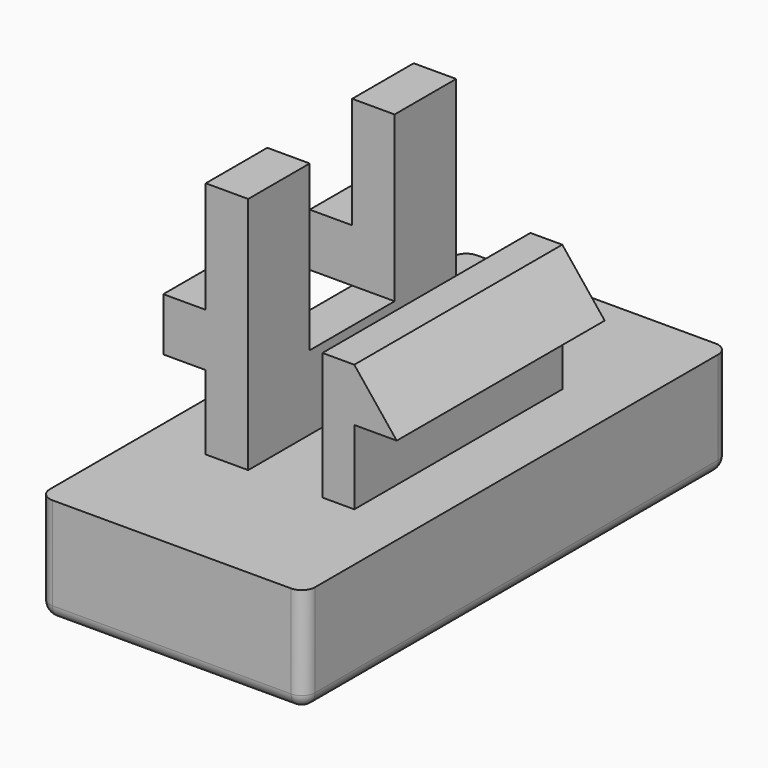
from build123d import *

# Parameters (mm, degrees)
F0_W      = 5
F0_H      = 10
F1_DEPTH  = 2
F2_R      = 0.25
F4_DEPTH  = 2.45
F5_W      = 0.8
F5_H      = 4.5
F6_DEPTH  = 2.45
F7_W      = 2
F7_H      = 3.1
F8_DEPTH  = 0.8
F9_W      = 1.45
F9_H      = 1
F10_DEPTH = 0.8


# Not quite as in the source:
# - a feature names something its author has since deleted; it is built from what else it names


with BuildPart() as f1:
    # F0 (on Top) → F1 (new body)
    with BuildSketch(Plane.XY):
        Rectangle(F0_W, F0_H)
    extrude(amount=F1_DEPTH)

    # F2
    f2_edges = [f1.edges().sort_by_distance(p)[0] for p in [
        (2.5, 5, 1),
        (-2.5, -5, 1),
        (0, 5, 0),
        (2.5, 0, 0),
        (-2.5, 0, 0),
        (0, -5, 0),
        (-2.5, 5, 1),
        (2.5, -5, 1),
    ]]
    fillet(f2_edges, radius=F2_R)

    # F3 (on Front) → F4 (join, symmetric)
    with BuildSketch(Plane.XZ):
        Polygon((0.8, 4.4), (0.8, 2), (1.4, 2), (1.4, 3.4), (2.2, 3.4), (1.4, 4.4), align=None)
    extrude(amount=F4_DEPTH, both=True)

    # F5 (on Front) → F6 (join, symmetric)
    with BuildSketch(Plane.XZ):
        with Locations((-1, 4.25)):
            Rectangle(F5_W, F5_H)
    extrude(amount=F6_DEPTH, both=True)

    # F7 (on face) → F8 (cut, through all)
    with BuildSketch(Plane(origin=(-1.4, 0, 0), x_dir=(0, -1, 0), z_dir=(-1, 0, 0))):
        with Locations((0, 4.95)):
            Rectangle(F7_W, F7_H)
    extrude(amount=-F8_DEPTH, mode=Mode.SUBTRACT)

    # F9 (on face) → F10 (join)
    with BuildSketch(Plane(origin=(-1.4, 0, 0), x_dir=(0, -1, 0), z_dir=(-1, 0, 0))):
        with Locations((-1.725, 3.9)):
            Rectangle(F9_W, F9_H)
        with Locations((1.725, 3.9)):
            Rectangle(F9_W, F9_H)
    extrude(amount=F10_DEPTH)


solid = f1.part
